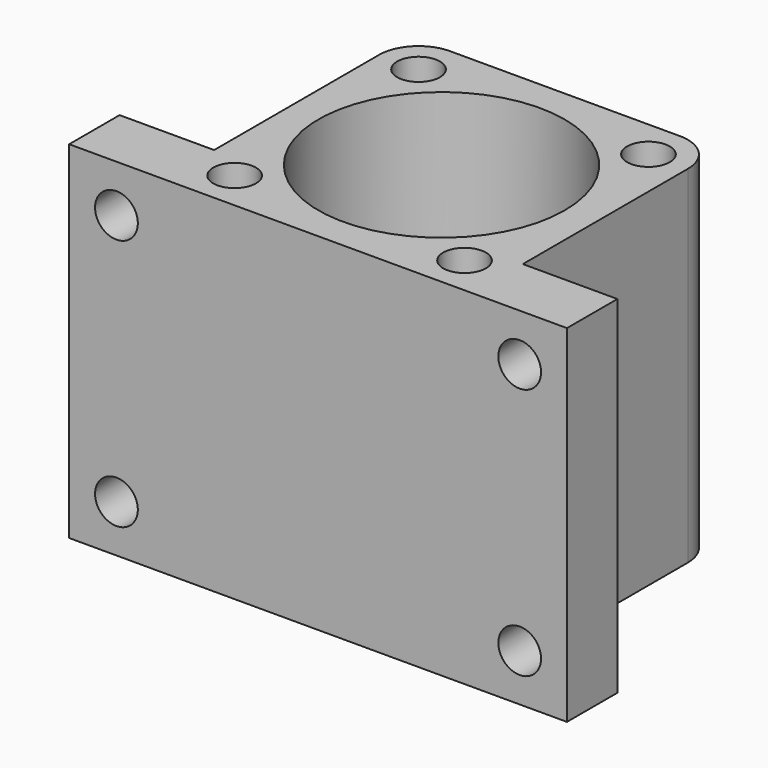
from build123d import *

# Parameters (mm, degrees)
F0_R     = 2.15265
F0_R_2   = 12.4079
F1_DEPTH = 30.8864
F2_R     = 2.15265
F2_R_2   = 12.4079
F2_R_3   = 10.8204
F3_DEPTH = 4.0386
F4_R     = 2.15265
F5_DEPTH = 6.35
F6_R     = 3.96875


with BuildPart() as f1:
    # F0 (on Top) → F1 (new body)
    with BuildSketch(Plane.XY):
        Polygon((15.5487902681, 15.5487902681), (-15.5487902681, 15.5487902681), (-15.5487902681, -9.1987902681), (-25.0737902681, -9.1987902681), (-25.0737902681, -15.5487902681), (25.0737902681, -15.5487902681), (25.0737902681, -9.1987902681), (15.5487902681, -9.1987902681), align=None)
        with Locations((-11.5800402681, -11.5800402681)):
            Circle(F0_R, mode=Mode.SUBTRACT)
        with Locations((11.5800402681, -11.5800402681)):
            Circle(F0_R, mode=Mode.SUBTRACT)
        with Locations((-11.5800402681, 11.5800402681)):
            Circle(F0_R, mode=Mode.SUBTRACT)
        Circle(F0_R_2, mode=Mode.SUBTRACT)
        with Locations((11.5800402681, 11.5800402681)):
            Circle(F0_R, mode=Mode.SUBTRACT)
    extrude(amount=F1_DEPTH)

    # F2 (on face) → F3 (join)
    with BuildSketch(Plane(origin=(0, 0, 0), x_dir=(1, 0, 0), z_dir=(0, 0, -1))):
        Polygon((-15.5487902681, -15.5487902681), (15.5487902681, -15.5487902681), (15.5487902681, 9.1987902681), (25.0737902681, 9.1987902681), (25.0737902681, 15.5487902681), (-25.0737902681, 15.5487902681), (-25.0737902681, 9.1987902681), (-15.5487902681, 9.1987902681), align=None)
        with Locations((-11.5800402681, -11.5800402681)):
            Circle(F2_R, mode=Mode.SUBTRACT)
        with Locations((11.5800402681, -11.5800402681)):
            Circle(F2_R, mode=Mode.SUBTRACT)
        with Locations((-11.5800402681, 11.5800402681)):
            Circle(F2_R, mode=Mode.SUBTRACT)
        Circle(F2_R_2, mode=Mode.SUBTRACT)
        with Locations((11.5800402681, 11.5800402681)):
            Circle(F2_R, mode=Mode.SUBTRACT)
        Circle(F2_R_2)
        Circle(F2_R_3, mode=Mode.SUBTRACT)
    extrude(amount=F3_DEPTH)

    # F4 (on face) → F5 (cut, through all)
    with BuildSketch(Plane(origin=(0, -9.1987902681, 0), x_dir=(-1, 0, 0), z_dir=(0, 1, 0))):
        with Locations((-20.3112902681, 0.7239)):
            Circle(F4_R)
        with Locations((-20.3112902681, 26.1239)):
            Circle(F4_R)
        with Locations((20.3112902681, 26.1239)):
            Circle(F4_R)
        with Locations((20.3112902681, 0.7239)):
            Circle(F4_R)
    extrude(amount=-F5_DEPTH, mode=Mode.SUBTRACT)

    # F6
    f6_edges = [f1.edges().sort_by_distance(p)[0] for p in [
        (-15.54879, 15.54879, 13.4239),
        (15.54879, 15.54879, 13.4239),
    ]]
    fillet(f6_edges, radius=F6_R)


solid = f1.part
